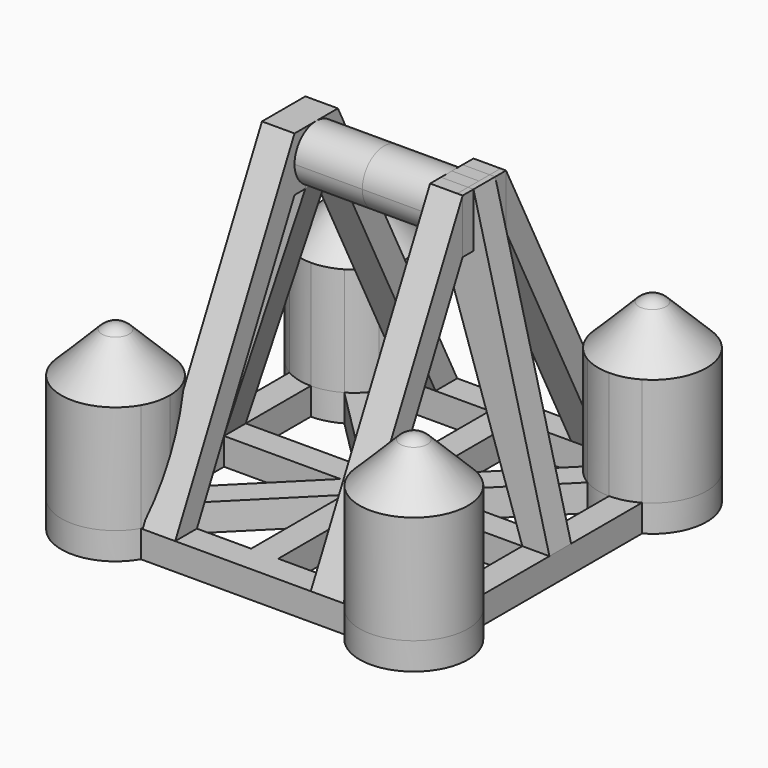
from build123d import *

# Parameters (mm, degrees)
F0_R           = 19.05
F1_DEPTH       = 12.7
F2_R           = 19.05
F3_DEPTH       = 50.8
F5_DEPTH       = 31.75
F7_DEPTH       = 12.7
F15_DEPTH      = 2.54
F15_DEPTH_BACK = 12.7
F18_W          = 25.4
F18_H          = 25.4
F19_DEPTH      = 2.54
F22_DEPTH      = 6.35


# Not quite as in the source:
# - after a boolean that leaves OpenCascade's solid faulty, fix() repairs it
# - a feature of the source that left no trace in its solid (it failed there, or was rolled back) is left out


with BuildPart() as f1:
    # F0 (on Top) → F1 (new body)
    with BuildSketch(Plane.XY):
        with BuildLine():
            Line((82.55, 6.35), (82.55, 47.8529547439))
            ThreePointArc((82.55, 47.8529547439), (87.8105122421, 87.8105122421), (47.8529547439, 82.55))
            Line((47.8529547439, 82.55), (0, 82.55))
            Line((0, 82.55), (-47.8529547439, 82.55))
            ThreePointArc((-47.8529547439, 82.55), (-87.8105122421, 87.8105122421), (-82.55, 47.8529547439))
            Line((-82.55, 47.8529547439), (-82.55, 6.35))
            Line((-82.55, 6.35), (-82.55, 0))
            Line((-82.55, 0), (-82.55, -6.35))
            Line((-82.55, -6.35), (-82.55, -47.8529547439))
            ThreePointArc((-82.55, -47.8529547439), (-87.8105122421, -87.8105122421), (-47.8529547439, -82.55))
            Line((-47.8529547439, -82.55), (0, -82.55))
            Line((0, -82.55), (47.8529547439, -82.55))
            ThreePointArc((47.8529547439, -82.55), (87.8105122421, -87.8105122421), (82.55, -47.8529547439))
            Line((82.55, -47.8529547439), (82.55, -6.35))
            Line((82.55, -6.35), (82.55, 0))
            Line((82.55, 0), (82.55, 6.35))
        make_face()
        with Locations((-69.85, -69.85)):
            Circle(F0_R, mode=Mode.SUBTRACT)
        with BuildLine():
            Line((-6.35, -69.85), (-44.45, -69.85))
            ThreePointArc((-44.45, -69.85), (-45.345713546, -63.1641982245), (-47.9696807387, -56.9499368597))
            Line((-47.9696807387, -56.9499368597), (-6.35, -15.3302561211))
            Line((-6.35, -15.3302561211), (-6.35, -69.85))
        make_face(mode=Mode.SUBTRACT)
        with BuildLine():
            Line((-69.85, -6.35), (-15.3302561211, -6.35))
            Line((-15.3302561211, -6.35), (-56.9499368597, -47.9696807387))
            ThreePointArc((-56.9499368597, -47.9696807387), (-63.1641982245, -45.345713546), (-69.85, -44.45))
            Line((-69.85, -44.45), (-69.85, -6.35))
        make_face(mode=Mode.SUBTRACT)
        with Locations((69.85, -69.85)):
            Circle(F0_R, mode=Mode.SUBTRACT)
        with BuildLine():
            ThreePointArc((47.9696807387, -56.9499368597), (45.345713546, -63.1641982245), (44.45, -69.85))
            Line((44.45, -69.85), (6.35, -69.85))
            Line((6.35, -69.85), (6.35, -15.3302561211))
            Line((6.35, -15.3302561211), (47.9696807387, -56.9499368597))
        make_face(mode=Mode.SUBTRACT)
        with BuildLine():
            Line((56.9499368597, -47.9696807387), (15.3302561211, -6.35))
            Line((15.3302561211, -6.35), (69.85, -6.35))
            Line((69.85, -6.35), (69.85, -44.45))
            ThreePointArc((69.85, -44.45), (63.1641982245, -45.345713546), (56.9499368597, -47.9696807387))
        make_face(mode=Mode.SUBTRACT)
        with BuildLine():
            Line((-56.9499368597, 47.9696807387), (-15.3302561211, 6.35))
            Line((-15.3302561211, 6.35), (-69.85, 6.35))
            Line((-69.85, 6.35), (-69.85, 44.45))
            ThreePointArc((-69.85, 44.45), (-63.1641982245, 45.345713546), (-56.9499368597, 47.9696807387))
        make_face(mode=Mode.SUBTRACT)
        with BuildLine():
            Line((-6.35, 69.85), (-6.35, 15.3302561211))
            Line((-6.35, 15.3302561211), (-47.9696807387, 56.9499368597))
            ThreePointArc((-47.9696807387, 56.9499368597), (-45.345713546, 63.1641982245), (-44.45, 69.85))
            Line((-44.45, 69.85), (-6.35, 69.85))
        make_face(mode=Mode.SUBTRACT)
        with Locations((-69.85, 69.85)):
            Circle(F0_R, mode=Mode.SUBTRACT)
        with BuildLine():
            Line((69.85, 6.35), (15.3302561211, 6.35))
            Line((15.3302561211, 6.35), (56.9499368597, 47.9696807387))
            ThreePointArc((56.9499368597, 47.9696807387), (63.1641982245, 45.345713546), (69.85, 44.45))
            Line((69.85, 44.45), (69.85, 6.35))
        make_face(mode=Mode.SUBTRACT)
        with BuildLine():
            Line((6.35, 15.3302561211), (6.35, 69.85))
            Line((6.35, 69.85), (44.45, 69.85))
            ThreePointArc((44.45, 69.85), (45.345713546, 63.1641982245), (47.9696807387, 56.9499368597))
            Line((47.9696807387, 56.9499368597), (6.35, 15.3302561211))
        make_face(mode=Mode.SUBTRACT)
        with Locations((69.85, 69.85)):
            Circle(F0_R, mode=Mode.SUBTRACT)
    extrude(amount=F1_DEPTH)

    # F2 (on face) → F3 (join)
    with BuildSketch(Plane.XY.offset(12.7)):
        with BuildLine():
            ThreePointArc((-69.85, -44.45), (-76.4240037456, -45.3154840123), (-82.55, -47.8529547439))
            ThreePointArc((-82.55, -47.8529547439), (-87.8105122421, -87.8105122421), (-47.8529547439, -82.55))
            ThreePointArc((-47.8529547439, -82.55), (-45.3154840123, -76.4240037456), (-44.45, -69.85))
            ThreePointArc((-44.45, -69.85), (-45.345713546, -63.1641982245), (-47.9696807387, -56.9499368597))
            ThreePointArc((-47.9696807387, -56.9499368597), (-51.8894877579, -51.8894877579), (-56.9499368597, -47.9696807387))
            ThreePointArc((-56.9499368597, -47.9696807387), (-63.1641982245, -45.345713546), (-69.85, -44.45))
        make_face()
        with Locations((-69.85, -69.85)):
            Circle(F2_R, mode=Mode.SUBTRACT)
        with BuildLine():
            ThreePointArc((95.25, 69.85), (76.4240037456, 94.3845159877), (47.8529547439, 82.55))
            ThreePointArc((47.8529547439, 82.55), (45.3154840123, 76.4240037456), (44.45, 69.85))
            ThreePointArc((44.45, 69.85), (45.345713546, 63.1641982245), (47.9696807387, 56.9499368597))
            ThreePointArc((47.9696807387, 56.9499368597), (51.8894877579, 51.8894877579), (56.9499368597, 47.9696807387))
            ThreePointArc((56.9499368597, 47.9696807387), (63.1641982245, 45.345713546), (69.85, 44.45))
            ThreePointArc((69.85, 44.45), (76.4240037456, 45.3154840123), (82.55, 47.8529547439))
            ThreePointArc((82.55, 47.8529547439), (91.8470452561, 57.15), (95.25, 69.85))
        make_face()
        with Locations((69.85, 69.85)):
            Circle(F2_R, mode=Mode.SUBTRACT)
    extrude(amount=F3_DEPTH)

    # F10 (on offset) → F11 (revolve)
    with BuildSketch(Plane.XZ.offset(69.85)):
        with BuildLine():
            Line((-76.2, 82.55), (-95.25, 63.5))
            Line((-95.25, 63.5), (-88.9, 63.5))
            Line((-88.9, 63.5), (-69.85, 82.55))
            Line((-69.85, 82.55), (-69.85, 85.1802561211))
            ThreePointArc((-69.85, 85.1802561211), (-73.2865952359, 84.496674827), (-76.2, 82.55))
        make_face()
    revolve(axis=Axis((-69.85, -69.85, 63.5), (0, 0, 1)))


with BuildPart() as f5:
    # F4 (on Right) → F5 (new body, symmetric)
    with BuildSketch(Plane.YZ):
        with BuildLine():
            ThreePointArc((0, 127), (8.9802561211, 130.7197438789), (12.7, 139.7))
            ThreePointArc((12.7, 139.7), (-8.9802561211, 148.6802561211), (0, 127))
        make_face()
    extrude(amount=F5_DEPTH, both=True)

    # F6 (on face) → F7 (join)
    with BuildSketch(Plane(origin=(-31.75, 0, 0), x_dir=(0, -1, 0), z_dir=(-1, 0, 0))):
        with BuildLine():
            ThreePointArc((1.818e-07, 152.4), (-8.9802560568, 148.6802561853), (-12.7, 139.7))
            ThreePointArc((-12.7, 139.7), (-8.9802561211, 130.7197438789), (0, 127))
            ThreePointArc((0, 127), (8.9802561211, 130.7197438789), (12.7, 139.7))
            ThreePointArc((12.7, 139.7), (8.9802561853, 148.6802560568), (1.818e-07, 152.4))
        make_face()
        with BuildLine():
            Line((-12.7, 152.4), (-12.7, 139.7))
            ThreePointArc((-12.7, 139.7), (-8.9802560568, 148.6802561853), (1.818e-07, 152.4))
            Line((1.818e-07, 152.4), (-12.7, 152.4))
        make_face()
        with BuildLine():
            ThreePointArc((0, 127), (-8.9802561211, 130.7197438789), (-12.7, 139.7))
            Line((-12.7, 139.7), (-12.7, 127))
            Line((-12.7, 127), (0, 127))
        make_face()
    extrude(amount=F7_DEPTH)

    # F8: F5 across plane


with BuildPart() as f5_1:
    add(f5.part)
    add(f5.part.mirror(Plane.YZ))


with BuildPart() as f12_1:
    # F12: instance of F1
    add(f1.part.mirror(Plane.XZ))


with BuildPart() as f1_1:
    add(f1.part)

    add(f12_1.part)  # F13 merges F12_1
    # F13: F1, F12_1 across plane
    add(f1.part.mirror(Plane.YZ))
    add(f12_1.part.mirror(Plane.YZ))

    add(f5_1.part)  # F15 merges F5
    # F14 (on face) → F15 (join, two sides)
    with BuildSketch(Plane(origin=(-44.45, 0, 0), x_dir=(0, -1, 0), z_dir=(-1, 0, 0))) as f15_sk:
        Polygon((12.7, 139.7), (12.7, 127), (69.85, 12.7), (82.55, 12.7), (12.7, 152.4), align=None)
    extrude(amount=F15_DEPTH)
    extrude(f15_sk.sketch, amount=-F15_DEPTH_BACK)

    add(f1_1.part.fix(), mode=Mode.REPLACE)


with BuildPart() as f16_1:
    # F16: instance of F1
    add(f1_1.part.mirror(Plane.YZ))


with BuildPart() as f1_2:
    add(f1_1.part)

    add(f16_1.part)  # F17 merges F16_1
    # F17: F1, F16_1 across plane
    add(f1_1.part.mirror(Plane.XZ))
    add(f16_1.part.mirror(Plane.XZ))

    # F18 (on face) → F19 (join)
    with BuildSketch(Plane(origin=(-44.45, 0, 0), x_dir=(0, -1, 0), z_dir=(-1, 0, 0))):
        with Locations((0, 139.7)):
            Rectangle(F18_W, F18_H)
    extrude(amount=F19_DEPTH)

    # F21 (on Front) → F22 (join, symmetric)
    with BuildSketch(Plane.XZ):
        Polygon((-31.75, 152.4), (-46.99, 152.4), (-82.55, 12.7), (-69.85, 12.7), (-31.75, 127), align=None)
    extrude(amount=F22_DEPTH, both=True)

    # F23: F1 across plane


with BuildPart() as f1_3:
    add(f1_2.part)
    add(f1_2.part.mirror(Plane.YZ))


solid = f1_3.part
